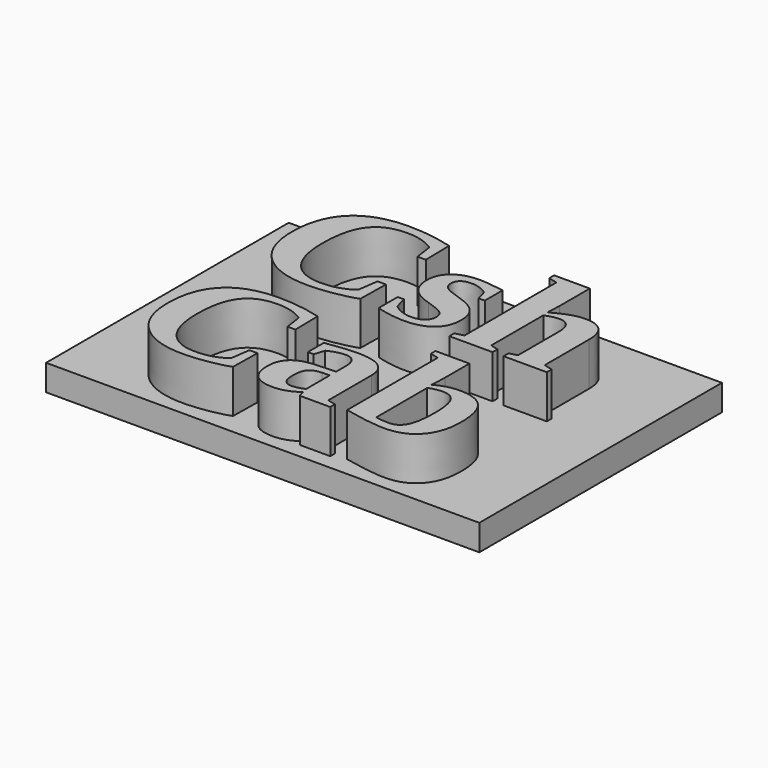
from build123d import *

# Parameters (mm, degrees)
F0_W         = 20
F0_H         = 14
F1_DEPTH     = 1.2
F2_TEXT_SIZE = 8.7463556851
F3_TEXT_SIZE = 8.3318868252
F4_DEPTH     = 2


# Not quite as in the source:
# - Text() gives the source's letters only with a copy of the font that has no kerning and outlines rounded to 1/6400 em; it was checked with that copy


with BuildPart() as f1:
    # F0 (on Top) → F1 (new body)
    with BuildSketch(Plane.XY):
        Rectangle(F0_W, F0_H)
    extrude(amount=F1_DEPTH)

    # F2 (on face) + F3 (on face) → F4 (join)
    with BuildSketch(Plane.XY.offset(1.2)):
        with Locations((-7.5, 0.7026239067)):
            Text('Csh', F2_TEXT_SIZE, font='Tinos', font_style=FontStyle.BOLD, text_align=(TextAlign.LEFT, TextAlign.BOTTOM))
    with BuildSketch(Plane.XY.offset(1.2)):
        with Locations((-7.5, -6.2963346074)):
            Text('Cab', F3_TEXT_SIZE, font='Tinos', font_style=FontStyle.BOLD, text_align=(TextAlign.LEFT, TextAlign.BOTTOM))
    extrude(amount=F4_DEPTH)


solid = f1.part
